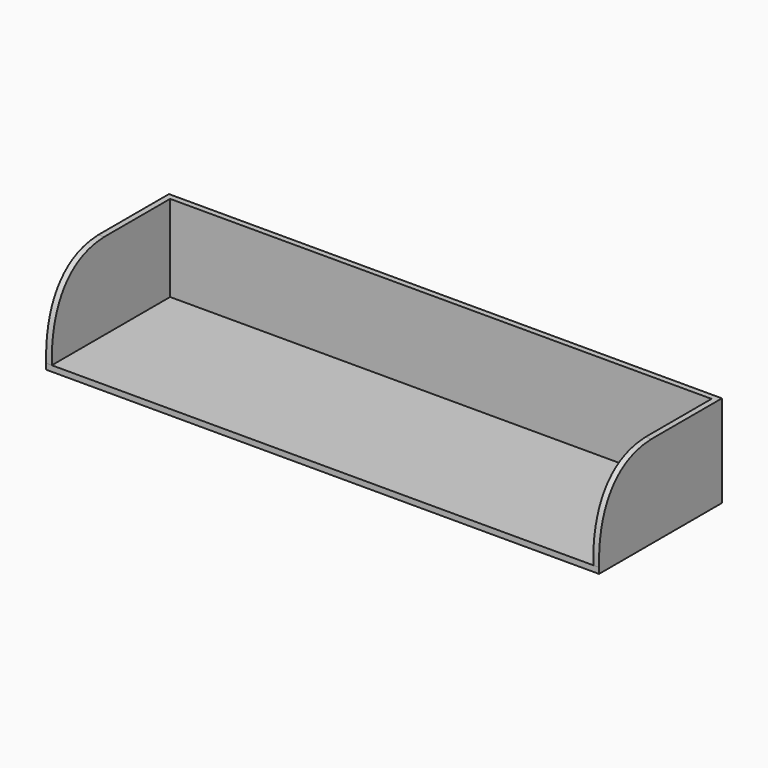
from build123d import *

# Parameters (mm, degrees)
F1_DEPTH = 1828.8
F3_DEPTH = 19.05
F5_DEPTH = 19.05


# Not quite as in the source:
# - the dataset's text gives a spline's control points without its knots; the knots are read off the source's solid


with BuildPart() as f1:
    # F0 (on Right) → F1 (new body)
    with BuildSketch(Plane.YZ):
        Polygon((-508, 0), (0, 0), (0, 304.8), (-19.05, 304.8), (-19.05, 19.05), (-508, 19.05), align=None)
    extrude(amount=F1_DEPTH)

    # F2 (on face) → F3 (join)
    with BuildSketch(Plane.YZ.offset(1828.8)):
        with BuildLine():
            Line((-508, 19.05), (-508, 0))
            Line((-508, 0), (0, 0))
            Line((0, 0), (0, 304.8))
            Line((0, 304.8), (-19.05, 304.8))
            Line((-19.05, 304.8), (-291.9989773071, 304.8))
            add(Edge.make_bspline(
                [(-291.9989773071, 304.8), (-492.9765110924, 298.0255581824), (-509.9911244928, 37.8132619011), (-507.4893097422, 43.3757593081), (-508, 19.05)],
                knots=[0, 0, 0, 0, 0.7436196079, 1, 1, 1, 1], degree=3))
        make_face()
    extrude(amount=-F3_DEPTH)

    # F4 (on face) → F5 (join)
    with BuildSketch(Plane(origin=(0, 0, 0), x_dir=(0, -1, 0), z_dir=(-1, 0, 0))):
        with BuildLine():
            Line((19.05, 304.8), (0, 304.8))
            Line((0, 304.8), (0, 0))
            Line((0, 0), (508, 0))
            Line((508, 0), (508, 19.05))
            add(Edge.make_bspline(
                [(291.9989773071, 304.8), (492.9765110924, 298.0255581824), (509.9911244928, 37.8132619011), (507.4893097422, 43.3757593081), (508, 19.05)],
                knots=[0, 0, 0, 0, 0.7436196079, 1, 1, 1, 1], degree=3))
            Line((291.9989773071, 304.8), (19.05, 304.8))
        make_face()
    extrude(amount=-F5_DEPTH)


solid = f1.part
